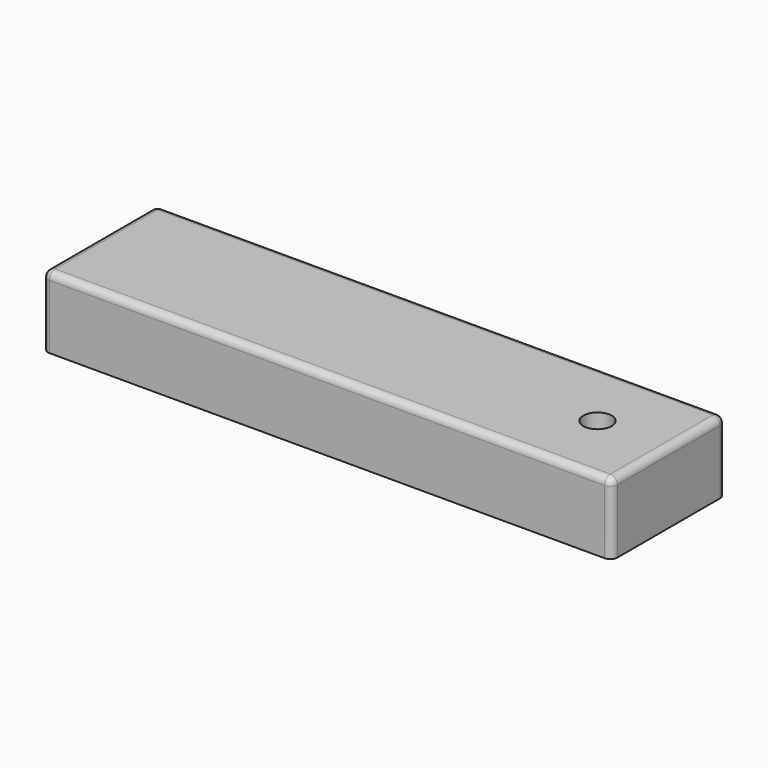
from build123d import *

# Parameters (mm, degrees)
F0_W         = 400
F0_H         = 100
F1_DEPTH     = 50
F2_R         = 5
F3_T1_DEPTH  = 57.5
F3_T3_DEPTH  = 90
F3_S7_W      = 5
F3_S7_H      = 5
F3_T8_DEPTH  = 5
F3_T12_ANGLE = 90
F4_R         = 10
F5_DEPTH     = 50.001


# Not quite as in the source:
# - a fillet or chamfer that OpenCascade refuses, or shapes differently, is made with other operations: its cross-section is extruded or revolved along the edge and cut away or added


with BuildPart() as f1:
    # F0 (on Top) → F1 (new body)
    with BuildSketch(Plane.XY):
        with Locations((-0.9229257703, 15.3983329495)):
            Rectangle(F0_W, F0_H)
    extrude(amount=F1_DEPTH)

    # F2
    f2_edges = [f1.edges().sort_by_distance(p)[0] for p in [
        (-200.922926, -34.601667, 25),
        (199.077074, -34.601667, 25),
        (199.077074, 65.398333, 25),
        (199.077074, 15.398333, 50),
        (-0.922926, -34.601667, 50),
        (-0.922926, 65.398333, 50),
    ]]
    fillet(f2_edges, radius=F2_R)

    # F3: fillet of radius 5 on 1 edges, made by hand

    # F3_s2 → F3_t1 (cut)
    with BuildSketch(Plane.XY.offset(-12.5)):
        with BuildLine():
            ThreePointArc((-195.9229257703, 65.3983329495), (-199.4584596762, 63.9338668555), (-200.9229257703, 60.3983329495))
            Line((-200.9229257703, 60.3983329495), (-200.9229257703, 65.3983329495))
            Line((-200.9229257703, 65.3983329495), (-195.9229257703, 65.3983329495))
        make_face()
    extrude(amount=F3_T1_DEPTH, mode=Mode.SUBTRACT)

    # F3_s4 → F3_t3 (cut)
    with BuildSketch(Plane.XZ.offset(-60.3983329495)):
        with BuildLine():
            ThreePointArc((-200.9229257703, 45), (-199.4584596762, 48.5355339059), (-195.9229257703, 50))
            Line((-195.9229257703, 50), (-200.9229257703, 50))
            Line((-200.9229257703, 50), (-200.9229257703, 45))
        make_face()
    extrude(amount=F3_T3_DEPTH, mode=Mode.SUBTRACT)


with BuildPart() as f3_tool6:
    # F3_s7 → F3_t8 (new body)
    with BuildSketch(Plane.YZ.offset(-195.9229257703)):
        with Locations((-32.1016670505, 47.5)):
            Rectangle(F3_S7_W, F3_S7_H)
    extrude(amount=-F3_T8_DEPTH)

    # F3_s9 → F3_t10 (revolve, cut)
    with BuildSketch(Plane(origin=(-195.9229257703, -29.6016670505, 45), x_dir=(0, 0.7071067812, -0.7071067812), z_dir=(0, 0.7071067812, 0.7071067812))):
        with BuildLine():
            ThreePointArc((0, -5), (5, 0), (0, 5))
            Line((0, 5), (0, -5))
        make_face()
    revolve(axis=Axis((-195.9229257703, -29.6016670505, 45), (-1, 0, 0)), mode=Mode.SUBTRACT)


with BuildPart() as f1_1:
    add(f1.part)

    # F3_t5: cut F3_tool6
    add(f3_tool6.part, mode=Mode.SUBTRACT)

    # F3_s11 → F3_t12 (revolve, cut)
    with BuildSketch(Plane.XY.offset(45)):
        with BuildLine():
            ThreePointArc((-200.9229257703, 60.3983329495), (-199.4584596762, 63.9338668555), (-195.9229257703, 65.3983329495))
            Line((-195.9229257703, 65.3983329495), (-200.9229257703, 65.3983329495))
            Line((-200.9229257703, 65.3983329495), (-200.9229257703, 60.3983329495))
        make_face()
    revolve(axis=Axis((-200.9229257703, 60.3983329495, 45), (1, 0, 0)), revolution_arc=F3_T12_ANGLE, mode=Mode.SUBTRACT)

    # F4 (on face) → F5 (cut, through all)
    with BuildSketch(Plane.XY.offset(50)):
        with Locations((149.0770742297, 15.3983329495)):
            Circle(F4_R)
    extrude(amount=-F5_DEPTH, mode=Mode.SUBTRACT)


solid = f1_1.part
